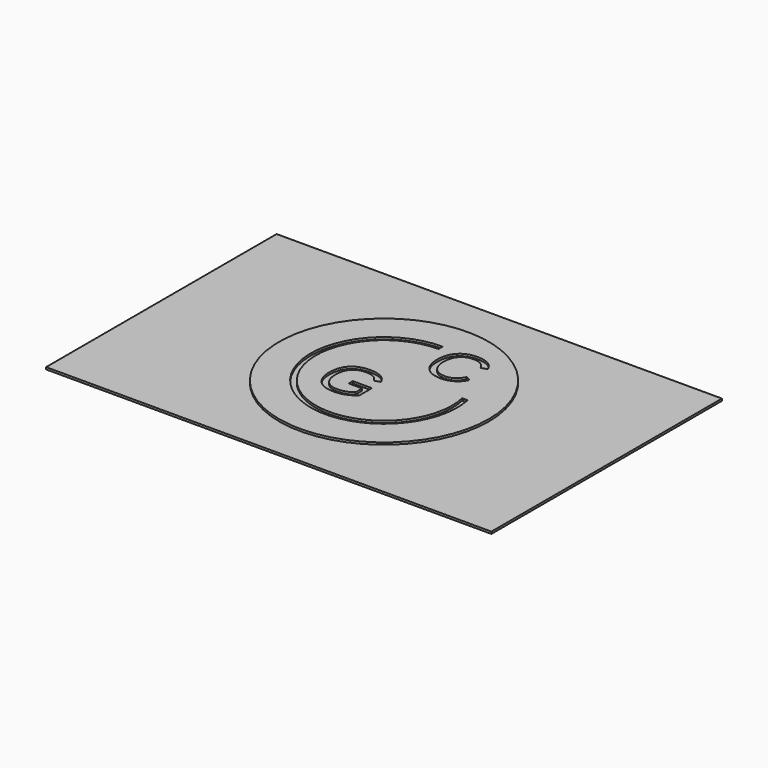
from build123d import *

# Parameters (mm, degrees)
F0_W     = 85
F0_H     = 55
F1_DEPTH = 0.4
F2_R     = 20
F3_DEPTH = 0.4


with BuildPart() as f1:
    # F0 (on Top) → F1 (new body)
    with BuildSketch(Plane.XY):
        Rectangle(F0_W, F0_H)
    extrude(amount=F1_DEPTH)

    # F2 (on face) → F3 (join)
    with BuildSketch(Plane.XY.offset(0.4)):
        Circle(F2_R)
        with BuildLine():
            add(Edge.make_bspline(
                [(-7.4961080118, -5.409697216), (-8.0117330118, -4.399931591), (-8.0117330118, -3.032744091)],
                knots=[0, 0, 0, 1, 1, 1], degree=2))
            add(Edge.make_bspline(
                [(-8.0117330118, -3.032744091), (-8.0117330118, -0.938994091), (-6.8886861368, 0.2084668465)],
                knots=[0, 0, 0, 1, 1, 1], degree=2))
            add(Edge.make_bspline(
                [(-6.8886861368, 0.2084668465), (-5.7656392618, 1.355927784), (-3.7324361368, 1.355927784)],
                knots=[0, 0, 0, 1, 1, 1], degree=2))
            add(Edge.make_bspline(
                [(-3.7324361368, 1.355927784), (-2.3047017618, 1.355927784), (-1.4140767618, 0.873505909)],
                knots=[0, 0, 0, 1, 1, 1], degree=2))
            add(Edge.make_bspline(
                [(-1.4140767618, 0.873505909), (-0.5234517618, 0.391084034), (-0.0410298868, -0.671415966)],
                knots=[0, 0, 0, 1, 1, 1], degree=2))
            Line((-0.0410298868, -0.671415966), (-1.1523580118, -0.999540966))
            add(Edge.make_bspline(
                [(-1.1523580118, -0.999540966), (-1.5175923868, -0.267119091), (-2.1611470743, 0.0678418465)],
                knots=[0, 0, 0, 1, 1, 1], degree=2))
            add(Edge.make_bspline(
                [(-2.1611470743, 0.0678418465), (-2.8047017618, 0.402802784), (-3.7636861368, 0.402802784)],
                knots=[0, 0, 0, 1, 1, 1], degree=2))
            add(Edge.make_bspline(
                [(-3.7636861368, 0.402802784), (-5.2539205118, 0.402802784), (-6.0410298868, -0.497587841)],
                knots=[0, 0, 0, 1, 1, 1], degree=2))
            add(Edge.make_bspline(
                [(-6.0410298868, -0.497587841), (-6.8281392618, -1.397978466), (-6.8281392618, -3.032744091)],
                knots=[0, 0, 0, 1, 1, 1], degree=2))
            add(Edge.make_bspline(
                [(-6.8281392618, -3.032744091), (-6.8281392618, -4.661650341), (-5.9922017618, -5.605009716)],
                knots=[0, 0, 0, 1, 1, 1], degree=2))
            add(Edge.make_bspline(
                [(-5.9922017618, -5.605009716), (-5.1562642618, -6.548369091), (-3.6777486368, -6.548369091)],
                knots=[0, 0, 0, 1, 1, 1], degree=2))
            add(Edge.make_bspline(
                [(-3.6777486368, -6.548369091), (-2.8359517618, -6.548369091), (-2.1064595743, -6.292509716)],
                knots=[0, 0, 0, 1, 1, 1], degree=2))
            add(Edge.make_bspline(
                [(-2.1064595743, -6.292509716), (-1.3769673868, -6.036650341), (-0.9257955118, -5.597197216)],
                knots=[0, 0, 0, 1, 1, 1], degree=2))
            Line((-0.9257955118, -5.597197216), (-0.9257955118, -4.046415966))
            Line((-0.9257955118, -4.046415966), (-3.4961080118, -4.046415966))
            Line((-3.4961080118, -4.046415966), (-3.4961080118, -3.069853466))
            Line((-3.4961080118, -3.069853466), (0.1484232382, -3.069853466))
            Line((0.1484232382, -3.069853466), (0.1484232382, -6.036650341))
            add(Edge.make_bspline(
                [(0.1484232382, -6.036650341), (-0.5351705118, -6.731962841), (-1.5273580118, -7.1137987785)],
                knots=[0, 0, 0, 1, 1, 1], degree=2))
            add(Edge.make_bspline(
                [(-1.5273580118, -7.1137987785), (-2.5195455118, -7.495634716), (-3.6777486368, -7.495634716)],
                knots=[0, 0, 0, 1, 1, 1], degree=2))
            add(Edge.make_bspline(
                [(-3.6777486368, -7.495634716), (-5.0273580118, -7.495634716), (-6.0039205118, -6.9575487785)],
                knots=[0, 0, 0, 1, 1, 1], degree=2))
            add(Edge.make_bspline(
                [(-6.0039205118, -6.9575487785), (-6.9804830118, -6.419462841), (-7.4961080118, -5.409697216)],
                knots=[0, 0, 0, 1, 1, 1], degree=2))
        make_face(mode=Mode.SUBTRACT)
        with BuildLine():
            ThreePointArc((13.716509354, 2.803100273), (-8.8531518731, -10.845353932), (0, 14))
            Line((0, 14), (0, 13))
            ThreePointArc((0, 13), (-8.1412436535, -10.135095055), (12.6941966607, 2.803100273))
            Line((12.6941966607, 2.803100273), (13.716509354, 2.803100273))
        make_face(mode=Mode.SUBTRACT)
        with BuildLine():
            add(Edge.make_bspline(
                [(7.744643158, 13.2869364135), (7.082533783, 13.6834207885), (6.172377533, 13.6834207885)],
                knots=[0, 0, 0, 1, 1, 1], degree=2))
            add(Edge.make_bspline(
                [(6.172377533, 13.6834207885), (4.744643158, 13.6834207885), (3.9506978455, 12.7654520385)],
                knots=[0, 0, 0, 1, 1, 1], degree=2))
            add(Edge.make_bspline(
                [(3.9506978455, 12.7654520385), (3.156752533, 11.8474832885), (3.156752533, 10.2478739135)],
                knots=[0, 0, 0, 1, 1, 1], degree=2))
            add(Edge.make_bspline(
                [(3.156752533, 10.2478739135), (3.156752533, 8.6677957885), (3.9839009705, 7.705881726)],
                knots=[0, 0, 0, 1, 1, 1], degree=2))
            add(Edge.make_bspline(
                [(3.9839009705, 7.705881726), (4.811049408, 6.7439676635), (6.221205658, 6.7439676635)],
                knots=[0, 0, 0, 1, 1, 1], degree=2))
            add(Edge.make_bspline(
                [(6.221205658, 6.7439676635), (8.027846283, 6.7439676635), (8.938002533, 8.5330301635)],
                knots=[0, 0, 0, 1, 1, 1], degree=2))
            Line((8.938002533, 8.5330301635), (9.889174408, 8.0564676635))
            add(Edge.make_bspline(
                [(9.889174408, 8.0564676635), (9.357924408, 6.9451395385), (8.396986908, 6.3650614135)],
                knots=[0, 0, 0, 1, 1, 1], degree=2))
            add(Edge.make_bspline(
                [(8.396986908, 6.3650614135), (7.436049408, 5.7849832885), (6.166518158, 5.7849832885)],
                knots=[0, 0, 0, 1, 1, 1], degree=2))
            add(Edge.make_bspline(
                [(6.166518158, 5.7849832885), (4.865736908, 5.7849832885), (3.916518158, 6.3259989135)],
                knots=[0, 0, 0, 1, 1, 1], degree=2))
            add(Edge.make_bspline(
                [(3.916518158, 6.3259989135), (2.967299408, 6.8670145385), (2.4702290955, 7.8709207885)],
                knots=[0, 0, 0, 1, 1, 1], degree=2))
            add(Edge.make_bspline(
                [(2.4702290955, 7.8709207885), (1.973158783, 8.8748270385), (1.973158783, 10.2478739135)],
                knots=[0, 0, 0, 1, 1, 1], degree=2))
            add(Edge.make_bspline(
                [(1.973158783, 10.2478739135), (1.973158783, 12.3045145385), (3.084486908, 13.4705301635)],
                knots=[0, 0, 0, 1, 1, 1], degree=2))
            add(Edge.make_bspline(
                [(3.084486908, 13.4705301635), (4.195815033, 14.6365457885), (6.160658783, 14.6365457885)],
                knots=[0, 0, 0, 1, 1, 1], degree=2))
            add(Edge.make_bspline(
                [(6.160658783, 14.6365457885), (7.533705658, 14.6365457885), (8.455580658, 14.0994364135)],
                knots=[0, 0, 0, 1, 1, 1], degree=2))
            add(Edge.make_bspline(
                [(8.455580658, 14.0994364135), (9.377455658, 13.5623270385), (9.811049408, 12.5056864135)],
                knots=[0, 0, 0, 1, 1, 1], degree=2))
            Line((9.811049408, 12.5056864135), (8.705580658, 12.1404520385))
            add(Edge.make_bspline(
                [(8.705580658, 12.1404520385), (8.406752533, 12.8904520385), (7.744643158, 13.2869364135)],
                knots=[0, 0, 0, 1, 1, 1], degree=2))
        make_face(mode=Mode.SUBTRACT)
    extrude(amount=F3_DEPTH)


solid = f1.part
